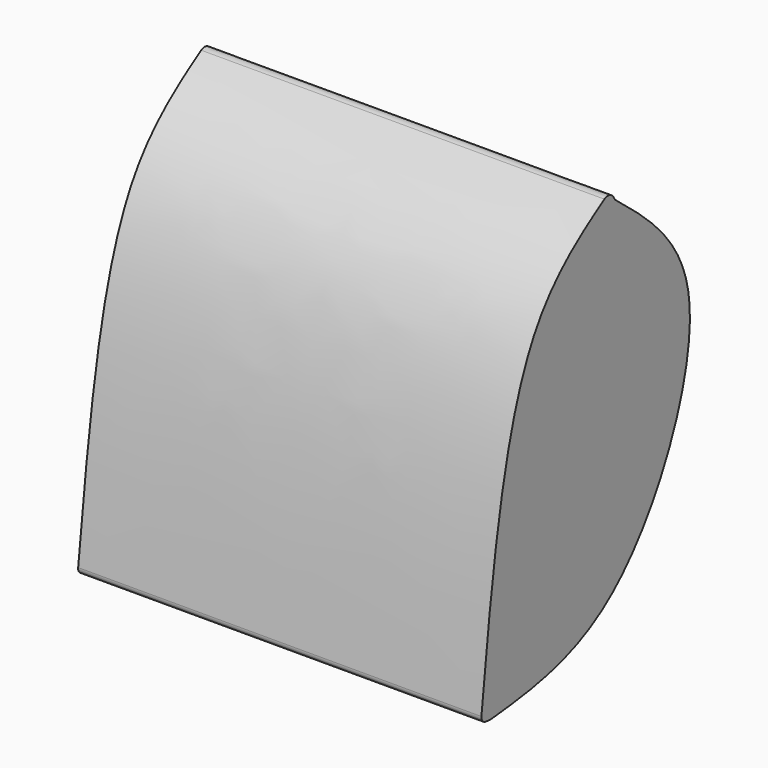
from build123d import *

# Parameters (mm, degrees)
F1_DEPTH    = 50
F0_R        = 1
F2_DEPTH    = 2
F3_DEPTH    = 5
F4_R        = 1
F5_T1_DEPTH = 50.1598643088


# Not quite as in the source:
# - a fillet or chamfer that OpenCascade refuses, or shapes differently, is made with other operations: its cross-section is extruded or revolved along the edge and cut away or added
# - the dataset's text gives a spline's control points without its knots; the knots are read off the source's solid


with BuildPart() as f1:
    # F0 (on Right) → F1 (new body)
    with BuildSketch(Plane.YZ):
        with BuildLine():
            add(Edge.make_bspline(
                [(0.0837637955, 0.7453579304), (1.7735396453, 15.7755371623), (4.6302666573, 40.2906845923), (15.6779868226, 47.2697126099), (20, 50)],
                knots=[0.0099623729, 0.0099623729, 0.0099623729, 0.0099623729, 0.6126842818, 1, 1, 1, 1], degree=3))
            ThreePointArc((0.0837637955, 0.7453579304), (0.2428246527, 0.1937865693), (0.7453267418, -0.0837435611))
            Line((0.7453267418, -0.0837435611), (1.4906204438, -0.1674834099))
            add(Edge.make_bspline(
                [(1.4906204438, -0.1674834099), (1.8408980596, 2.9500252166), (2.5403677843, 9.1748166807), (3.7447129168, 18.1359673406), (5.006656653, 24.9964443194), (6.2431372221, 29.9379404399), (7.299479719, 33.3233721789), (8.2978294113, 35.8365388722), (9.1713397017, 37.6393355352), (10.0939609865, 39.291765961), (11.3532120899, 41.1089550964), (13.0130694593, 42.9772264755), (14.8066337423, 44.6067327942), (17.3532343359, 46.5520549205), (19.4062531069, 47.8506885385), (20.8011142545, 48.7318454545)],
                knots=[0, 0, 0, 0, 0.125, 0.25, 0.375, 0.4375, 0.5, 0.5625, 0.59375, 0.625, 0.6875, 0.75, 0.8125, 0.875, 1, 1, 1, 1], degree=3))
            Line((20.8011142545, 48.7318454545), (20, 50))
        make_face()
    extrude(amount=-F1_DEPTH)

    # F0 (on Right) → F2 (join)
    with BuildSketch(Plane.YZ):
        with BuildLine():
            add(Edge.make_bspline(
                [(20.8011142545, 48.7318454545), (26.0719723661, 44.5220613355), (37.8958312253, 35.0784579987), (23.1198602378, 2.060703258), (8.2440899918, 0.5282410332), (1.4906204438, -0.1674834099)],
                knots=[0, 0, 0, 0, 0.3051589819, 0.6845482568, 1, 1, 1, 1], degree=3))
            add(Edge.make_bspline(
                [(1.4906204438, -0.1674834099), (1.8408980596, 2.9500252166), (2.5403677843, 9.1748166807), (3.7447129168, 18.1359673406), (5.006656653, 24.9964443194), (6.2431372221, 29.9379404399), (7.299479719, 33.3233721789), (8.2978294113, 35.8365388722), (9.1713397017, 37.6393355352), (10.0939609865, 39.291765961), (11.3532120899, 41.1089550964), (13.0130694593, 42.9772264755), (14.8066337423, 44.6067327942), (17.3532343359, 46.5520549205), (19.4062531069, 47.8506885385), (20.8011142545, 48.7318454545)],
                knots=[0, 0, 0, 0, 0.125, 0.25, 0.375, 0.4375, 0.5, 0.5625, 0.59375, 0.625, 0.6875, 0.75, 0.8125, 0.875, 1, 1, 1, 1], degree=3))
        make_face()
        with Locations((21.8817591667, 22.5125644356)):
            Circle(F0_R, mode=Mode.SUBTRACT)
        with Locations((21.8817591667, 22.5125644356)):
            Circle(F0_R)
    extrude(amount=-F2_DEPTH)

    # F0 (on Right) → F3 (join)
    with BuildSketch(Plane.YZ):
        with Locations((21.8817591667, 22.5125644356)):
            Circle(F0_R)
    extrude(amount=-F3_DEPTH)

    # F4
    f4_edges = [f1.edges().sort_by_distance(p)[0] for p in [
        (-25, 20, 50),
    ]]
    fillet(f4_edges, radius=F4_R)

    # F5: fillet of radius 1 on 1 edges, made by hand

    # F5_s2 → F5_t1 (cut)
    with BuildSketch(Plane.YZ.offset(-52.1598643088)):
        with BuildLine():
            ThreePointArc((20.534512705, 49.153872606), (20.4209287984, 48.6499443621), (20.0710179281, 48.2699346758))
            Line((20.0710179281, 48.2699346758), (20.081732389, 48.2530468007))
            ThreePointArc((20.081732389, 48.2530468007), (20.4466443036, 48.4841647223), (20.8117957779, 48.7149367272))
            Line((20.8117957779, 48.7149367272), (20.8180229817, 48.7425269779))
            ThreePointArc((20.8180229817, 48.7425269779), (20.684722207, 48.9535405536), (20.5544970614, 49.1546634894))
            Line((20.5544970614, 49.1546634894), (20.534512705, 49.153872606))
        make_face()
    extrude(amount=F5_T1_DEPTH, mode=Mode.SUBTRACT)


solid = f1.part
